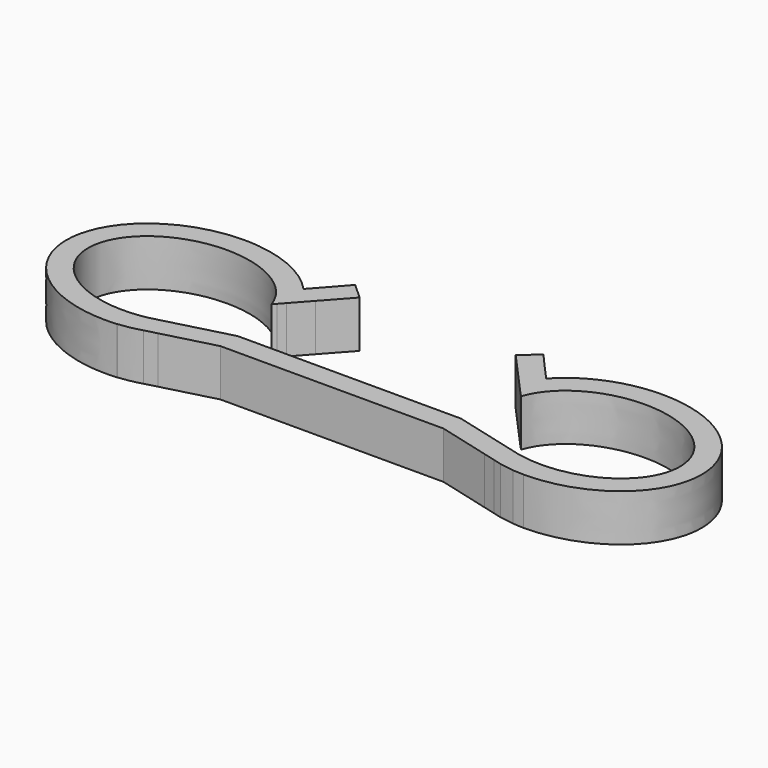
from build123d import *

# Parameters (mm, degrees)
F1_DEPTH = 6.5


# Not quite as in the source:
# - ends of sketch curves that miss each other by under 0.0002 mm in the source are joined


with BuildPart() as f1:
    # F0 (on Top) → F1 (new body)
    with BuildSketch(Plane.XY):
        with BuildLine():
            Line((-15.4360572198, 0), (0, 0))
            Line((0, 0), (15.4360572198, 0))
            Line((15.4360572198, 0), (22.5785540972, -1.8753532969))
            Line((22.5785540972, -1.8753532969), (24.2372755143, -2.3108716782))
            Line((24.2372755143, -2.3108716782), (25.4360572198, -2.6256270449))
            add(Edge.make_bspline(
                [(25.4360572198, -2.6256270449), (26.409631126, -2.8409522067), (27.4090879072, -2.9350034665)],
                knots=[4.4605481479, 4.4605481479, 4.4605481479, 4.6038126101, 4.6038126101, 4.6038126101], degree=2, weights=[1, 0.9974355086, 1]))
            add(Edge.make_bspline(
                [(27.4090879072, -2.9350034665), (28.1671167574, -3.0063357838), (28.9296869951, -3.0067787163)],
                knots=[4.6038126101, 4.6038126101, 4.6038126101, 4.7125491946, 4.7125491946, 4.7125491946], degree=2, weights=[1, 0.9985224084, 1]))
            add(Edge.make_bspline(
                [(28.9296869951, -3.0067787163), (53.4311857774, -3.0210094859), (42.3108067868, 14.4412975805), (31.1904277962, 31.903604647), (16.7916403321, 16.0535704123)],
                knots=[4.7125009223, 4.7125009223, 4.7125009223, 6.754819691, 6.754819691, 8.7971384597, 8.7971384597, 8.7971384597], degree=2, weights=[1, 0.522377679, 1, 0.522377679, 1]))
            Line((16.7916403321, 16.0535704123), (16.1451111023, 16.7724215104))
            Line((16.1451111023, 16.7724215104), (15.9389197568, 17.0016777735))
            Line((15.9389197568, 17.0016777735), (14.7280874781, 18.3479558272))
            Line((14.7280874781, 18.3479558272), (13.025946407, 20.2828743527))
            Line((13.025946407, 20.2828743527), (10.7953902187, 18.2767290214))
            Line((10.7953902187, 18.2767290214), (16.1451111023, 12.3285791857))
            Line((16.1451111023, 12.3285791857), (16.8643018326, 11.528938547))
            Line((16.8643018326, 11.528938547), (17.2680627309, 11.127852488))
            add(Edge.make_bspline(
                [(25.4360572198, 0.3836022246), (54.3204678279, -6.2097181263), (39.370508439, 13.4555871478), (24.4205490501, 33.1208924219), (17.2680627309, 11.127852488)],
                knots=[4.4164574814, 4.4164574814, 4.4164574814, 6.8009375444, 6.8009375444, 9.1854176074, 9.1854176074, 9.1854176074], degree=2, weights=[1, 0.3695793658, 1, 0.3695793658, 1]))
            Line((25.4360572198, 0.3836022246), (15.4360572198, 3))
            Line((15.4360572198, 3), (0, 3))
            Line((0, 3), (-15.2705321592, 3))
            Line((-15.2705321592, 3), (-15.4360572198, 3))
            Line((-15.4360572198, 3), (-16.0547256122, 2.8381317394))
            Line((-16.0547256122, 2.8381317394), (-17.1087004648, 2.5623699935))
            Line((-17.1087004648, 2.5623699935), (-25.4360572198, 0.3836022246))
            add(Edge.make_bspline(
                [(-17.2680627309, 11.127852488), (-24.4205490501, 33.1208924219), (-39.370508439, 13.4555871478), (-54.3204678279, -6.2097181263), (-25.4360572198, 0.3836022246)],
                knots=[3.380953007, 3.380953007, 3.380953007, 5.76543307, 5.76543307, 8.149913133, 8.149913133, 8.149913133], degree=2, weights=[1, 0.3695793658, 1, 0.3695793658, 1]))
            Line((-17.2680627309, 11.127852488), (-16.8643018326, 11.528938547))
            Line((-16.8643018326, 11.528938547), (-16.1451111023, 12.3285791857))
            Line((-16.1451111023, 12.3285791857), (-14.013543256, 14.6985878667))
            Line((-14.013543256, 14.6985878667), (-10.7953902187, 18.2767290214))
            Line((-10.7953902187, 18.2767290214), (-13.025946407, 20.2828743527))
            Line((-13.025946407, 20.2828743527), (-14.7280874781, 18.3479558272))
            Line((-14.7280874781, 18.3479558272), (-15.8682951869, 17.0802025288))
            Line((-15.8682951869, 17.0802025288), (-15.9389197568, 17.0016777735))
            Line((-15.9389197568, 17.0016777735), (-16.1451111023, 16.7724215104))
            Line((-16.1451111023, 16.7724215104), (-16.7916406562, 16.0535700519))
            add(Edge.make_bspline(
                [(-16.7916406562, 16.0535700519), (-21.285689854, 21.0005729952), (-28.9329279759, 20.9999984796)],
                knots=[3.7692321546, 3.7692321546, 3.7692321546, 4.7116446629, 4.7116446629, 4.7116446629], degree=2, weights=[1, 0.8910213437, 1]))
            add(Edge.make_bspline(
                [(-28.9329279759, 20.9999984796), (-28.9344906831, 21.0000002986), (-28.9360533902, 21)],
                knots=[4.7115507193, 4.7115507193, 4.7115507193, 4.711773769, 4.711773769, 4.711773769], degree=2, weights=[1, 0.9999999938, 1]))
            add(Edge.make_bspline(
                [(-28.9360533902, 21), (-44.7308001421, 20.9961812437), (-43.9263336329, 8.3816232809), (-43.1218671236, -4.232934682), (-27.4090674102, -2.9441350843)],
                knots=[4.7118528883, 4.7118528883, 4.7118528883, 6.3336037978, 6.3336037978, 7.9553547073, 7.9553547073, 7.9553547073], degree=2, weights=[1, 0.6888640882, 1, 0.6888640882, 1]))
            Line((-27.4090674102, -2.9441350843), (-27.3359285804, -2.927950861))
            add(Edge.make_bspline(
                [(-27.3359285804, -2.927950861), (-25.7454911542, -2.7710392295), (-24.2372755143, -2.3108716782)],
                knots=[1.6846261213, 1.6846261213, 1.6846261213, 1.9121420834, 1.9121420834, 1.9121420834], degree=2, weights=[1, 0.9935365356, 1]))
            Line((-24.2372755143, -2.3108716782), (-22.5785540972, -1.8753532969))
            Line((-22.5785540972, -1.8753532969), (-15.4360572198, 0))
        make_face()
    extrude(amount=F1_DEPTH)


solid = f1.part
